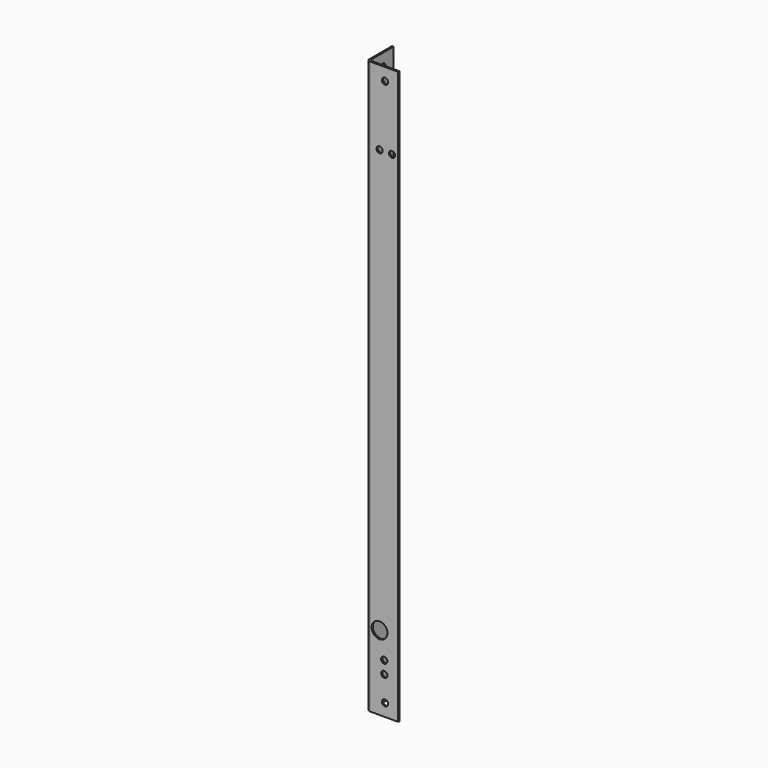
from build123d import *

# Parameters (mm, degrees)
F1_DEPTH    = 584.2
F2_T1_DEPTH = 584.2
F2_T3_DEPTH = 600.075
F3_R        = 3.175
F4_DEPTH    = 1.5875
F5_R        = 3.175
F6_DEPTH    = 1.5875
F7_R        = 3.175
F8_DEPTH    = 1.5875
F9_R        = 3.175
F10_DEPTH   = 1.5875
F11_R       = 8.0645
F12_DEPTH   = 1.5875


# Not quite as in the source:
# - a fillet or chamfer that OpenCascade refuses, or shapes differently, is made with other operations: its cross-section is extruded or revolved along the edge and cut away or added


with BuildPart() as f1:
    # F0 (on Top) → F1 (new body)
    with BuildSketch(Plane.XY):
        Polygon((-5.119352553, 3.4975720825), (-5.119352553, 33.6600720825), (-6.706852553, 33.6600720825), (-6.706852553, 1.9100720825), (25.043147447, 1.9100720825), (25.043147447, 3.4975720825), align=None)
    extrude(amount=F1_DEPTH)

    # F2: fillet of radius 3.175 on 2 edges, made by hand

    # F2_s2 → F2_t1 (join)
    with BuildSketch(Plane.XY):
        with BuildLine():
            add(Edge.make_bspline(
                [(-1.944352553, 3.4975720825), (-5.119352553, 3.4975720825), (-5.119352553, 6.6725720825)],
                knots=[0, 0, 0, 1, 1, 1], degree=2, weights=[1, 1, 1]))
            Line((-5.119352553, 6.6725720825), (-5.119352553, 3.4975720825))
            Line((-5.119352553, 3.4975720825), (-1.944352553, 3.4975720825))
        make_face()
    extrude(amount=F2_T1_DEPTH)

    # F2_s4 → F2_t3 (cut)
    with BuildSketch(Plane.XY.offset(-7.9375)):
        with BuildLine():
            add(Edge.make_bspline(
                [(-6.706852553, 5.0850720825), (-6.706852553, 1.9100720825), (-3.531852553, 1.9100720825)],
                knots=[0, 0, 0, 1, 1, 1], degree=2, weights=[1, 1, 1]))
            Line((-3.531852553, 1.9100720825), (-6.706852553, 1.9100720825))
            Line((-6.706852553, 1.9100720825), (-6.706852553, 5.0850720825))
        make_face()
    extrude(amount=F2_T3_DEPTH, mode=Mode.SUBTRACT)

    # F3 (on face) → F4 (cut)
    with BuildSketch(Plane.YZ.offset(-5.119352553)):
        with Locations((20.1663220825, 12.7)):
            Circle(F3_R)
        with Locations((20.1663220825, 571.5)):
            Circle(F3_R)
    extrude(amount=-F4_DEPTH, mode=Mode.SUBTRACT)

    # F5 (on face) → F6 (cut)
    with BuildSketch(Plane(origin=(0, 3.4975720825, 0), x_dir=(-1, 0, 0), z_dir=(0, 1, 0))):
        with Locations((-11.549397447, 12.7)):
            Circle(F5_R)
        with Locations((-11.549397447, 571.5)):
            Circle(F5_R)
    extrude(amount=-F6_DEPTH, mode=Mode.SUBTRACT)

    # F7 (on face) → F8 (cut)
    with BuildSketch(Plane.XZ.offset(-1.9100720825)):
        with Locations((5.993147447, 508)):
            Circle(F7_R)
        with Locations((18.693147447, 508)):
            Circle(F7_R)
    extrude(amount=-F8_DEPTH, mode=Mode.SUBTRACT)

    # F9 (on face) → F10 (cut)
    with BuildSketch(Plane.XZ.offset(-1.9100720825)):
        with Locations((10.755647447, 38.1)):
            Circle(F9_R)
        with Locations((10.755647447, 50.8)):
            Circle(F9_R)
    extrude(amount=-F10_DEPTH, mode=Mode.SUBTRACT)

    # F11 (on face) → F12 (cut)
    with BuildSketch(Plane.XZ.offset(-1.9100720825)):
        with Locations((5.993147447, 76.2)):
            Circle(F11_R)
    extrude(amount=-F12_DEPTH, mode=Mode.SUBTRACT)


solid = f1.part
